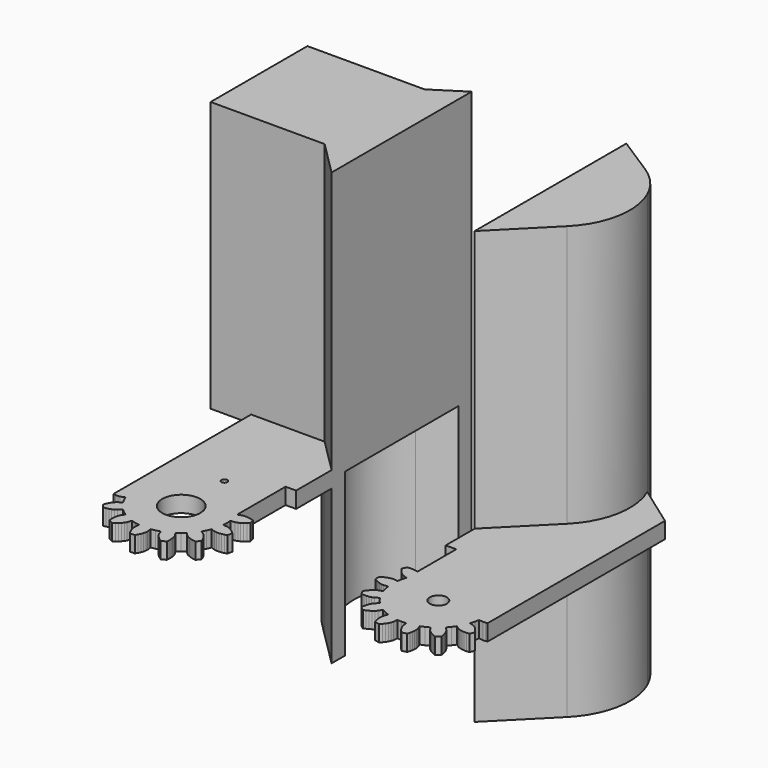
from build123d import *

# Parameters (mm, degrees)
F1_DEPTH = 1.5
F0_R     = 1.6
F2_DEPTH = 50
F3_DEPTH = 30


# Not quite as in the source:
# - ends of sketch curves that miss each other by under 0.0002 mm in the source are joined


with BuildPart() as f1:
    # F0 (on Top) → F1 (new body, symmetric)
    with BuildSketch(Plane.XY):
        Polygon((-12.6828804, -37.9996929195), (-11.8884367355, -38.2222305677), (-11.8880267366, -38.2224279172), (-11.075543, -38.3664943195), (-11.1792258, -39.1773131195), (-11.1500412, -39.5862277195), (-11.049381, -40.0020257195), (-10.8967016, -40.4206431195), (-10.6978958, -40.8390065195), (-10.4565196, -41.2543727195), (-9.5434404, -41.2543727195), (-9.302115, -40.8390065195), (-9.1033092, -40.4206431195), (-8.950579, -40.0020257195), (-8.8499188, -39.5862277195), (-8.820785, -39.1773131195), (-8.9244678, -38.3664943195), (-8.1119840634, -38.2224279172), (-8.1115408, -38.2223493195), (-7.3171558, -37.9996929195), (-7.0589394, -38.7751549195), (-6.8550028, -39.1308311195), (-6.5838324, -39.4619201195), (-6.2647068, -39.7727145195), (-5.9041792, -40.0633667195), (-5.5066184, -40.3329369195), (-4.6838108, -39.9365445195), (-4.646549, -39.4578053195), (-4.6491144, -38.9947125195), (-4.693031, -38.5513555195), (-4.7828454, -38.1327635195), (-4.9339246, -37.7516365195), (-5.3789072, -37.0664715195), (-4.7096916266, -36.5840362135), (-4.709287, -36.5837445195), (-4.0899842, -36.0385589195), (-3.5209988, -36.6249941195), (-3.1831534, -36.8570993195), (-2.7948636, -37.0377695195), (-2.3725632, -37.1791713195), (-1.9218148, -37.2846829195), (-1.4464538, -37.3550663195), (-0.8770112, -36.6409453195), (-1.0512806, -36.1933973195), (-1.2544552, -35.7773199195), (-1.4865096, -35.3969041195), (-1.7489424, -35.0588555195), (-2.0504658, -34.7809287195), (-2.7488388, -34.3565455195), (-2.3551745142, -33.6315615111), (-2.3549356, -33.6311215195), (-2.0336002, -32.8714075195), (-1.2662154, -33.1527887195), (-0.86106, -33.2152727195), (-0.4331716, -33.2096847195), (0.0087884, -33.1539317195), (0.4607052, -33.0533223195), (0.9195562, -32.9104727195), (1.1227562, -32.0200757195), (0.7714742, -31.6924411195), (0.4079494, -31.4057259195), (0.033782, -31.1636639195), (-0.3494024, -30.9728083195), (-0.741426, -30.8533775195), (-1.5548356, -30.7739771195), (-1.5148031909, -29.9499745831), (-1.5147798, -29.9494931195), (-1.5548356, -29.1254663195), (-0.741426, -29.0460913195), (-0.3494024, -28.9266605195), (0.033782, -28.7358049195), (0.4079494, -28.4937683195), (0.7714742, -28.2070531195), (1.1227562, -27.8793931195), (0.9195562, -26.9889961195), (0.4607052, -26.8461465195), (0.0087884, -26.7455371195), (-0.4331716, -26.6898095195), (-0.86106, -26.6842215195), (-1.2662154, -26.7467055195), (-1.999996, -27.0157423195), (-1.999996, -15.8072914928), (-0.05, -15.8072914928), (-0.05, -8.999886363), (-7.8088611939, -1.2753778), (-20.002250767, -1.2753778), (-20.0087992, -33.1539317195), (-19.5667884, -33.2096847195), (-19.1389, -33.2152727195), (-18.7337954, -33.1527887195), (-17.9664106, -32.8714075195), (-17.6450069939, -33.6311141557), (-17.6448212, -33.6315533195), (-17.251172, -34.3565455195), (-17.9495196, -34.7809287195), (-18.2510684, -35.0588555195), (-18.5134504, -35.3969041195), (-18.745581, -35.7773199195), (-18.9487302, -36.1933973195), (-19.1229996, -36.6409453195), (-18.5535062, -37.3550663195), (-18.078196, -37.2846829195), (-17.6274476, -37.1791713195), (-17.2051218, -37.0377695195), (-16.8168066, -36.8570993195), (-16.479012, -36.6249941195), (-15.9100012, -36.0385589195), (-15.2906723648, -36.583686083), (-15.2903174, -36.5839985195), (-14.6211036, -37.0664715195), (-15.0660862, -37.7516365195), (-15.2171654, -38.1327635195), (-15.306929, -38.5513555195), (-15.3509218, -38.9947125195), (-15.3534618, -39.4578053195), (-15.3162, -39.9365445195), (-14.493367, -40.3329369195), (-14.0958062, -40.0633667195), (-13.735304, -39.7727145195), (-13.4161784, -39.4619201195), (-13.1449572, -39.1308311195), (-12.9410968, -38.7751549195), align=None)
        with BuildLine():
            ThreePointArc((-9.99998, -26.4247471195), (-7.5074285963, -27.4571957159), (-6.47498, -29.9497471195))
            ThreePointArc((-6.47498, -29.9497471195), (-12.4925314037, -32.4422985232), (-9.99998, -26.4247471195))
        make_face(mode=Mode.SUBTRACT)
        with BuildLine():
            ThreePointArc((-9.4549722, -19.9497471195), (-9.6146012888, -20.3351258307), (-9.99998, -20.4947549195))
            ThreePointArc((-9.99998, -20.4947549195), (-10.3853587112, -19.5643684084), (-9.4549722, -19.9497471195))
        make_face(mode=Mode.SUBTRACT)
        Polygon((-6.3914999282, -1.2753778), (-7.8088611939, -1.2753778), (-0.05, -8.999886363), (-0.05, -7.5888005143), align=None)
        Polygon((-8.4115295291, -0.6753778), (-7.8088611939, -1.2753778), (-6.3914999282, -1.2753778), (-6.9941682635, -0.6753778), align=None)
        with BuildLine():
            Line((-20.0019887813, 0), (-20.0021275162, -0.6753778))
            Line((-20.0021275162, -0.6753778), (-8.4115295291, -0.6753778))
            Line((-8.4115295291, -0.6753778), (-6.9941682635, -0.6753778))
            Line((-6.9941682635, -0.6753778), (-8.8192027426, 1.1415762748))
            ThreePointArc((-8.8192027426, 1.1415762748), (-11.5431807788, 5.203648739), (-12.5000003164, 10))
            Line((-12.5000003164, 10), (-15.0591228454, 10))
            Line((-15.0591228454, 10), (-20.0019887813, 0))
        make_face()
        with BuildLine():
            Line((-12.1022985118, 15.9820039061), (-15.0591228454, 10))
            Line((-15.0591228454, 10), (-12.5000003164, 10))
            ThreePointArc((-12.5000003164, 10), (-11.8911847625, 13.8535351113), (-10.1240431199, 17.331695494))
            Line((-10.1240431199, 17.331695494), (-12.1022985118, 15.9820039061))
        make_face()
        Polygon((-20.0021275162, -0.6753778), (-20.002250767, -1.2753778), (-7.8088611939, -1.2753778), (-8.4115295291, -0.6753778), align=None)
    extrude(amount=F1_DEPTH, both=True)



with BuildPart() as f1b:
    # F0 (on Top) → F1, piece 2 (new body, symmetric)
    with BuildSketch(Plane.XY):
        with BuildLine():
            Line((45.5568809356, -32.5242657195), (45.7794119864, -31.729845607))
            Line((45.7794119864, -31.729845607), (45.7796203111, -31.7294128346))
            Line((45.7796203111, -31.7294128346), (45.9237077356, -30.9169283195))
            Line((45.9237077356, -30.9169283195), (46.7345011356, -31.0206111195))
            Line((46.7345011356, -31.0206111195), (47.1434157356, -30.9914519195))
            Line((47.1434157356, -30.9914519195), (47.5068643356, -30.9034663195))
            Line((47.5068643356, -30.9034663195), (47.5068643356, 10.1083564))
            Line((47.5068643356, 10.1083564), (39.8461772472, 15.5849402666))
            ThreePointArc((39.8461772472, 15.5849402666), (40.7766908436, 7.6257287323), (37.0316684565, 0.541259019))
            Line((37.0316684565, 0.541259019), (27.5569297356, -8.9911811067))
            Line((27.5569297356, -8.9911811067), (27.5569297356, -15.6989350928))
            Line((27.5569297356, -15.6989350928), (29.5069257356, -15.6989350928))
            Line((29.5069257356, -15.6989350928), (29.5069257356, -24.6967985195))
            Line((29.5069257356, -24.6967985195), (29.3238933356, -24.6242561195))
            Line((29.3238933356, -24.6242561195), (28.9053267356, -24.5344163195))
            Line((28.9053267356, -24.5344163195), (28.4619443356, -24.4904997195))
            Line((28.4619443356, -24.4904997195), (27.9988769356, -24.4879343195))
            Line((27.9988769356, -24.4879343195), (27.5201123356, -24.5252215195))
            Line((27.5201123356, -24.5252215195), (27.1237453356, -25.3480037195))
            Line((27.1237453356, -25.3480037195), (27.3933155356, -25.7455645195))
            Line((27.3933155356, -25.7455645195), (27.6839931356, -26.1060921195))
            Line((27.6839931356, -26.1060921195), (27.9947367356, -26.4252177195))
            Line((27.9947367356, -26.4252177195), (28.3259019356, -26.6964135195))
            Line((28.3259019356, -26.6964135195), (28.6815781356, -26.9003247195))
            Line((28.6815781356, -26.9003247195), (29.4569385356, -27.1585411195))
            Line((29.4569385356, -27.1585411195), (29.2345090358, -27.9529612023))
            Line((29.2345090358, -27.9529612023), (29.2343837356, -27.9534087195))
            Line((29.2343837356, -27.9534087195), (29.0901625356, -28.7658785195))
            Line((29.0901625356, -28.7658785195), (28.2793183356, -28.6621957195))
            Line((28.2793183356, -28.6621957195), (27.8704545356, -28.6913041195))
            Line((27.8704545356, -28.6913041195), (27.4546819356, -28.7919643195))
            Line((27.4546819356, -28.7919643195), (27.0360137356, -28.9447199195))
            Line((27.0360137356, -28.9447199195), (26.6177011356, -29.1435003195))
            Line((26.6177011356, -29.1435003195), (26.2023095356, -29.3848257195))
            Line((26.2023095356, -29.3848257195), (26.2023095356, -30.2979303195))
            Line((26.2023095356, -30.2979303195), (26.6177011356, -30.5392811195))
            Line((26.6177011356, -30.5392811195), (27.0360137356, -30.7380869195))
            Line((27.0360137356, -30.7380869195), (27.4546819356, -30.8907917195))
            Line((27.4546819356, -30.8907917195), (27.8704545356, -30.9914519195))
            Line((27.8704545356, -30.9914519195), (28.2793183356, -31.0206111195))
            Line((28.2793183356, -31.0206111195), (29.0901625356, -30.9169283195))
            Line((29.0901625356, -30.9169283195), (29.2343007326, -31.7294128446))
            Line((29.2343007326, -31.7294128446), (29.2343837356, -31.7298807195))
            Line((29.2343837356, -31.7298807195), (29.4569385356, -32.5242657195))
            Line((29.4569385356, -32.5242657195), (28.6815781356, -32.7824821195))
            Line((28.6815781356, -32.7824821195), (28.3259019356, -32.9863679195))
            Line((28.3259019356, -32.9863679195), (27.9947367356, -33.2575891195))
            Line((27.9947367356, -33.2575891195), (27.6839931356, -33.5766893195))
            Line((27.6839931356, -33.5766893195), (27.3933155356, -33.9371915195))
            Line((27.3933155356, -33.9371915195), (27.1237453356, -34.3347523195))
            Line((27.1237453356, -34.3347523195), (27.5201123356, -35.1575853195))
            Line((27.5201123356, -35.1575853195), (27.9988769356, -35.1948725195))
            Line((27.9988769356, -35.1948725195), (28.4619443356, -35.1923071195))
            Line((28.4619443356, -35.1923071195), (28.9053267356, -35.1483397195))
            Line((28.9053267356, -35.1483397195), (29.3238933356, -35.0585507195))
            Line((29.3238933356, -35.0585507195), (29.7050457356, -34.9074715195))
            Line((29.7050457356, -34.9074715195), (30.3902107356, -34.4624889195))
            Line((30.3902107356, -34.4624889195), (30.8726460484, -35.1317298871))
            Line((30.8726460484, -35.1317298871), (30.8729377356, -35.1321345195))
            Line((30.8729377356, -35.1321345195), (31.4180979356, -35.7513865195))
            Line((31.4180979356, -35.7513865195), (30.8316881356, -36.3203973195))
            Line((30.8316881356, -36.3203973195), (30.5995829356, -36.6582173195))
            Line((30.5995829356, -36.6582173195), (30.4189127356, -37.0465071195))
            Line((30.4189127356, -37.0465071195), (30.2775109356, -37.4688583195))
            Line((30.2775109356, -37.4688583195), (30.1719993356, -37.9196067195))
            Line((30.1719993356, -37.9196067195), (30.1016159356, -38.3949169195))
            Line((30.1016159356, -38.3949169195), (30.8157369356, -38.9643849195))
            Line((30.8157369356, -38.9643849195), (31.2632849356, -38.7901155195))
            Line((31.2632849356, -38.7901155195), (31.6793623356, -38.5869663195))
            Line((31.6793623356, -38.5869663195), (32.0597527356, -38.3548611195))
            Line((32.0597527356, -38.3548611195), (32.3978267356, -38.0924537195))
            Line((32.3978267356, -38.0924537195), (32.6757535356, -37.7909049195))
            Line((32.6757535356, -37.7909049195), (33.1001367356, -37.0925827195))
            Line((33.1001367356, -37.0925827195), (33.8251420267, -37.4861824058))
            Line((33.8251420267, -37.4861824058), (33.8255607356, -37.4864097195))
            Line((33.8255607356, -37.4864097195), (34.5852747356, -37.8077959195))
            Line((34.5852747356, -37.8077959195), (34.3038935356, -38.5752061195))
            Line((34.3038935356, -38.5752061195), (34.2414095356, -38.9803107195))
            Line((34.2414095356, -38.9803107195), (34.2469975356, -39.4081737195))
            Line((34.2469975356, -39.4081737195), (34.3027505356, -39.8501845195))
            Line((34.3027505356, -39.8501845195), (34.4033599356, -40.3021267195))
            Line((34.4033599356, -40.3021267195), (34.5461841356, -40.7609777195))
            Line((34.5461841356, -40.7609777195), (35.4366065356, -40.9641777195))
            Line((35.4366065356, -40.9641777195), (35.7642411356, -40.6128957195))
            Line((35.7642411356, -40.6128957195), (36.0509563356, -40.2493201195))
            Line((36.0509563356, -40.2493201195), (36.2929929356, -39.8751781195))
            Line((36.2929929356, -39.8751781195), (36.4838739356, -39.4919429195))
            Line((36.4838739356, -39.4919429195), (36.6033047356, -39.0999955195))
            Line((36.6033047356, -39.0999955195), (36.6826797356, -38.2865605195))
            Line((36.6826797356, -38.2865605195), (37.5067076121, -38.3265941598))
            Line((37.5067076121, -38.3265941598), (37.5071637356, -38.3266163195))
            Line((37.5071637356, -38.3266163195), (38.3311651356, -38.2865605195))
            Line((38.3311651356, -38.2865605195), (38.4105909356, -39.0999955195))
            Line((38.4105909356, -39.0999955195), (38.5299963356, -39.4919429195))
            Line((38.5299963356, -39.4919429195), (38.7208773356, -39.8751781195))
            Line((38.7208773356, -39.8751781195), (38.9629139356, -40.2493201195))
            Line((38.9629139356, -40.2493201195), (39.2496291356, -40.6128957195))
            Line((39.2496291356, -40.6128957195), (39.5772891356, -40.9641777195))
            Line((39.5772891356, -40.9641777195), (40.4676861356, -40.7609777195))
            Line((40.4676861356, -40.7609777195), (40.6105103356, -40.3021267195))
            Line((40.6105103356, -40.3021267195), (40.7111451356, -39.8501845195))
            Line((40.7111451356, -39.8501845195), (40.7668727356, -39.4081737195))
            Line((40.7668727356, -39.4081737195), (40.7724607356, -38.9803107195))
            Line((40.7724607356, -38.9803107195), (40.7099767356, -38.5752061195))
            Line((40.7099767356, -38.5752061195), (40.4285955356, -37.8077959195))
            Line((40.4285955356, -37.8077959195), (41.1883021717, -37.4863923134))
            Line((41.1883021717, -37.4863923134), (41.1887413356, -37.4862065195))
            Line((41.1887413356, -37.4862065195), (41.9137335356, -37.0925827195))
            Line((41.9137335356, -37.0925827195), (42.3381421356, -37.7909049195))
            Line((42.3381421356, -37.7909049195), (42.6160435356, -38.0924537195))
            Line((42.6160435356, -38.0924537195), (42.9541175356, -38.3548611195))
            Line((42.9541175356, -38.3548611195), (43.3345079356, -38.5869663195))
            Line((43.3345079356, -38.5869663195), (43.7505853356, -38.7901155195))
            Line((43.7505853356, -38.7901155195), (44.1981333356, -38.9643849195))
            Line((44.1981333356, -38.9643849195), (44.9122543356, -38.3949169195))
            Line((44.9122543356, -38.3949169195), (44.8418709356, -37.9196067195))
            Line((44.8418709356, -37.9196067195), (44.7363593356, -37.4688583195))
            Line((44.7363593356, -37.4688583195), (44.5949575356, -37.0465071195))
            Line((44.5949575356, -37.0465071195), (44.4142873356, -36.6582173195))
            Line((44.4142873356, -36.6582173195), (44.1821821356, -36.3203973195))
            Line((44.1821821356, -36.3203973195), (43.5957723356, -35.7513865195))
            Line((43.5957723356, -35.7513865195), (44.1408615089, -35.1320720054))
            Line((44.1408615089, -35.1320720054), (44.1411865356, -35.1317027195))
            Line((44.1411865356, -35.1317027195), (44.6236595356, -34.4624889195))
            Line((44.6236595356, -34.4624889195), (45.3088245356, -34.9074715195))
            Line((45.3088245356, -34.9074715195), (45.6899769356, -35.0585507195))
            Line((45.6899769356, -35.0585507195), (46.1085435356, -35.1483397195))
            Line((46.1085435356, -35.1483397195), (46.5519259356, -35.1923071195))
            Line((46.5519259356, -35.1923071195), (47.0149933356, -35.1948725195))
            Line((47.0149933356, -35.1948725195), (47.4937325356, -35.1575853195))
            Line((47.4937325356, -35.1575853195), (47.8901249356, -34.3347523195))
            Line((47.8901249356, -34.3347523195), (47.6205547356, -33.9371915195))
            Line((47.6205547356, -33.9371915195), (47.3299025356, -33.5766893195))
            Line((47.3299025356, -33.5766893195), (47.0191335356, -33.2575891195))
            Line((47.0191335356, -33.2575891195), (46.6880191356, -32.9863679195))
            Line((46.6880191356, -32.9863679195), (46.3323429356, -32.7824821195))
            Line((46.3323429356, -32.7824821195), (45.5568809356, -32.5242657195))
        make_face()
        with Locations((37.5069097356, -29.8413907195)):
            Circle(F0_R, mode=Mode.SUBTRACT)
    extrude(amount=F1_DEPTH, both=True)



with BuildPart() as f2:
    # F0 (on Top) → F2 (new body)
    with BuildSketch(Plane.XY):
        with BuildLine():
            Line((-8.8192027426, 1.1415762748), (-6.9941682635, -0.6753778))
            Line((-6.9941682635, -0.6753778), (-0.05, -4.5405198881))
            Line((-0.05, -4.5405198881), (-7.28327834, 3.1477115777))
            ThreePointArc((-7.28327834, 3.1477115777), (-9.9219987158, 11.2465718924), (-5.3618740808, 18.4409896542))
            Line((-5.3618740808, 18.4409896542), (-0.05, 21.8151911543))
            Line((-0.05, 21.8151911543), (-6.7420944452, 20.5258809799))
            ThreePointArc((-6.7420944452, 20.5258809799), (-8.5829688524, 19.0874998536), (-10.1240431199, 17.331695494))
            ThreePointArc((-10.1240431199, 17.331695494), (-11.8911847625, 13.8535351113), (-12.5000003164, 10))
            ThreePointArc((-12.5000003164, 10), (-11.5431807788, 5.203648739), (-8.8192027426, 1.1415762748))
        make_face()
        Polygon((-5.8053634872, 21.1258809799), (-6.7420944452, 20.5258809799), (-0.05, 21.8151911543), (-0.05, 22.999886363), (-0.05, 24.8123376548), align=None)
        Polygon((-6.9941682635, -0.6753778), (-6.3914999282, -1.2753778), (-0.05, -7.5888005143), (-0.05, -5.999886363), (-0.05, -4.5405198881), align=None)
        with BuildLine():
            Line((-7.28327834, 3.1477115777), (-0.05, -4.5405198881))
            Line((-0.05, -4.5405198881), (-0.05, 21.8151911543))
            Line((-0.05, 21.8151911543), (-5.3618740808, 18.4409896542))
            ThreePointArc((-5.3618740808, 18.4409896542), (-9.9219987158, 11.2465718924), (-7.28327834, 3.1477115777))
        make_face()
        with BuildLine():
            ThreePointArc((-17.0059758203, 20.5258809799), (-19.2368888885, 15.4716989952), (-19.9999346, 10))
            Line((-19.9999346, 10), (-15.0591228454, 10))
            Line((-15.0591228454, 10), (-12.1022985118, 15.9820039061))
            Line((-12.1022985118, 15.9820039061), (-10.1240431199, 17.331695494))
            ThreePointArc((-10.1240431199, 17.331695494), (-8.5829688524, 19.0874998536), (-6.7420944452, 20.5258809799))
            Line((-6.7420944452, 20.5258809799), (-17.0059758203, 20.5258809799))
        make_face()
        with BuildLine():
            Line((-27.5000003164, 10), (-19.9999346, 10))
            ThreePointArc((-19.9999346, 10), (-19.2368888885, 15.4716989952), (-17.0059758203, 20.5258809799))
            Line((-17.0059758203, 20.5258809799), (-27.5000003164, 20.5258809799))
            Line((-27.5000003164, 20.5258809799), (-27.5000003164, 10))
        make_face()
        Polygon((-27.5000003164, -0.6753778), (-20.0021275162, -0.6753778), (-20.0019887813, 0), (-19.9999346, 10), (-27.5000003164, 10), align=None)
        Polygon((-19.9999346, 10), (-20.0019887813, 0), (-15.0591228454, 10), align=None)
        with BuildLine():
            Line((-20.0019887813, 0), (-20.0021275162, -0.6753778))
            Line((-20.0021275162, -0.6753778), (-8.4115295291, -0.6753778))
            Line((-8.4115295291, -0.6753778), (-6.9941682635, -0.6753778))
            Line((-6.9941682635, -0.6753778), (-8.8192027426, 1.1415762748))
            ThreePointArc((-8.8192027426, 1.1415762748), (-11.5431807788, 5.203648739), (-12.5000003164, 10))
            Line((-12.5000003164, 10), (-15.0591228454, 10))
            Line((-15.0591228454, 10), (-20.0019887813, 0))
        make_face()
        with BuildLine():
            Line((-12.1022985118, 15.9820039061), (-15.0591228454, 10))
            Line((-15.0591228454, 10), (-12.5000003164, 10))
            ThreePointArc((-12.5000003164, 10), (-11.8911847625, 13.8535351113), (-10.1240431199, 17.331695494))
            Line((-10.1240431199, 17.331695494), (-12.1022985118, 15.9820039061))
        make_face()
        with BuildLine():
            ThreePointArc((-16.6196316573, 21.1258809799), (-16.8154800574, 20.82760428), (-17.0059758203, 20.5258809799))
            Line((-17.0059758203, 20.5258809799), (-6.7420944452, 20.5258809799))
            Line((-6.7420944452, 20.5258809799), (-5.8053634872, 21.1258809799))
            Line((-5.8053634872, 21.1258809799), (-16.6196316573, 21.1258809799))
        make_face()
        with BuildLine():
            Line((-27.5000003164, 20.5258809799), (-17.0059758203, 20.5258809799))
            ThreePointArc((-17.0059758203, 20.5258809799), (-16.8154800574, 20.82760428), (-16.6196316573, 21.1258809799))
            Line((-16.6196316573, 21.1258809799), (-27.5000003164, 21.1258809799))
            Line((-27.5000003164, 21.1258809799), (-27.5000003164, 20.5258809799))
        make_face()
        Polygon((-8.4115295291, -0.6753778), (-7.8088611939, -1.2753778), (-6.3914999282, -1.2753778), (-6.9941682635, -0.6753778), align=None)
        Polygon((-20.0021275162, -0.6753778), (-20.002250767, -1.2753778), (-7.8088611939, -1.2753778), (-8.4115295291, -0.6753778), align=None)
        Polygon((-27.5000003164, -1.2753778), (-20.002250767, -1.2753778), (-20.0021275162, -0.6753778), (-27.5000003164, -0.6753778), align=None)
    extrude(amount=F2_DEPTH)


with BuildPart() as f2b:
    # F0 (on Top) → F2, piece 2 (new body)
    with BuildSketch(Plane.XY):
        with BuildLine():
            Line((33.4049912244, 19.3934450196), (27.5569297356, 23.108242763))
            Line((27.5569297356, 23.108242763), (27.5569297356, 21.9235484419))
            Line((27.5569297356, 21.9235484419), (32.868804218, 18.5493466866))
            ThreePointArc((32.868804218, 18.5493466866), (37.4289291947, 11.3549283858), (34.7902086212, 3.2560674644))
            Line((34.7902086212, 3.2560674644), (27.5569297356, -4.4321645815))
            Line((27.5569297356, -4.4321645815), (27.5569297356, -5.891529963))
            Line((27.5569297356, -5.891529963), (35.5185359096, 2.5708391355))
            ThreePointArc((35.5185359096, 2.5708391355), (38.421128323, 11.4795854816), (33.4049912244, 19.3934450196))
        make_face()
        with BuildLine():
            ThreePointArc((37.0316684565, 0.541259019), (40.7766908436, 7.6257287323), (39.8461772472, 15.5849402666))
            ThreePointArc((39.8461772472, 15.5849402666), (37.7499815665, 18.9020978784), (34.788391552, 21.4763075705))
            Line((34.788391552, 21.4763075705), (27.5569297356, 26.108242763))
            Line((27.5569297356, 26.108242763), (27.5569297356, 23.108242763))
            Line((27.5569297356, 23.108242763), (33.4049912244, 19.3934450196))
            ThreePointArc((33.4049912244, 19.3934450196), (38.421128323, 11.4795854816), (35.5185359096, 2.5708391355))
            Line((35.5185359096, 2.5708391355), (27.5569297356, -5.891529963))
            Line((27.5569297356, -5.891529963), (27.5569297356, -8.9911811067))
            Line((27.5569297356, -8.9911811067), (37.0316684565, 0.541259019))
        make_face()
        with BuildLine():
            Line((32.868804218, 18.5493466866), (27.5569297356, 21.9235484419))
            Line((27.5569297356, 21.9235484419), (27.5569297356, -4.4321645815))
            Line((27.5569297356, -4.4321645815), (34.7902086212, 3.2560674644))
            ThreePointArc((34.7902086212, 3.2560674644), (37.4289291947, 11.3549283858), (32.868804218, 18.5493466866))
        make_face()
    extrude(amount=F2_DEPTH)


with BuildPart() as f1_1:
    add(f1.part)

    add(f2.part)  # F3 merges F2
    # F0 (on Top) → F3 (join)
    with BuildSketch(Plane.XY):
        with BuildLine():
            Line((-8.8192027426, 1.1415762748), (-6.9941682635, -0.6753778))
            Line((-6.9941682635, -0.6753778), (-0.05, -4.5405198881))
            Line((-0.05, -4.5405198881), (-7.28327834, 3.1477115777))
            ThreePointArc((-7.28327834, 3.1477115777), (-9.9219987158, 11.2465718924), (-5.3618740808, 18.4409896542))
            Line((-5.3618740808, 18.4409896542), (-0.05, 21.8151911543))
            Line((-0.05, 21.8151911543), (-6.7420944452, 20.5258809799))
            ThreePointArc((-6.7420944452, 20.5258809799), (-8.5829688524, 19.0874998536), (-10.1240431199, 17.331695494))
            ThreePointArc((-10.1240431199, 17.331695494), (-11.8911847625, 13.8535351113), (-12.5000003164, 10))
            ThreePointArc((-12.5000003164, 10), (-11.5431807788, 5.203648739), (-8.8192027426, 1.1415762748))
        make_face()
        Polygon((-6.9941682635, -0.6753778), (-6.3914999282, -1.2753778), (-0.05, -7.5888005143), (-0.05, -5.999886363), (-0.05, -4.5405198881), align=None)
        Polygon((-5.8053634872, 21.1258809799), (-6.7420944452, 20.5258809799), (-0.05, 21.8151911543), (-0.05, 22.999886363), (-0.05, 24.8123376548), align=None)
    extrude(amount=-F3_DEPTH)


with BuildPart() as f1b_1:
    add(f1b.part)

    add(f2b.part)  # F3#2 merges F2b
    # F0 (on Top) → F3, piece 2 (join)
    with BuildSketch(Plane.XY):
        with BuildLine():
            Line((33.4049912244, 19.3934450196), (27.5569297356, 23.108242763))
            Line((27.5569297356, 23.108242763), (27.5569297356, 21.9235484419))
            Line((27.5569297356, 21.9235484419), (32.868804218, 18.5493466866))
            ThreePointArc((32.868804218, 18.5493466866), (37.4289291947, 11.3549283858), (34.7902086212, 3.2560674644))
            Line((34.7902086212, 3.2560674644), (27.5569297356, -4.4321645815))
            Line((27.5569297356, -4.4321645815), (27.5569297356, -5.891529963))
            Line((27.5569297356, -5.891529963), (35.5185359096, 2.5708391355))
            ThreePointArc((35.5185359096, 2.5708391355), (38.421128323, 11.4795854816), (33.4049912244, 19.3934450196))
        make_face()
        with BuildLine():
            ThreePointArc((37.0316684565, 0.541259019), (40.7766908436, 7.6257287323), (39.8461772472, 15.5849402666))
            ThreePointArc((39.8461772472, 15.5849402666), (37.7499815665, 18.9020978784), (34.788391552, 21.4763075705))
            Line((34.788391552, 21.4763075705), (27.5569297356, 26.108242763))
            Line((27.5569297356, 26.108242763), (27.5569297356, 23.108242763))
            Line((27.5569297356, 23.108242763), (33.4049912244, 19.3934450196))
            ThreePointArc((33.4049912244, 19.3934450196), (38.421128323, 11.4795854816), (35.5185359096, 2.5708391355))
            Line((35.5185359096, 2.5708391355), (27.5569297356, -5.891529963))
            Line((27.5569297356, -5.891529963), (27.5569297356, -8.9911811067))
            Line((27.5569297356, -8.9911811067), (37.0316684565, 0.541259019))
        make_face()
    extrude(amount=-F3_DEPTH)


solid = Compound([f1_1.part, f1b_1.part])
